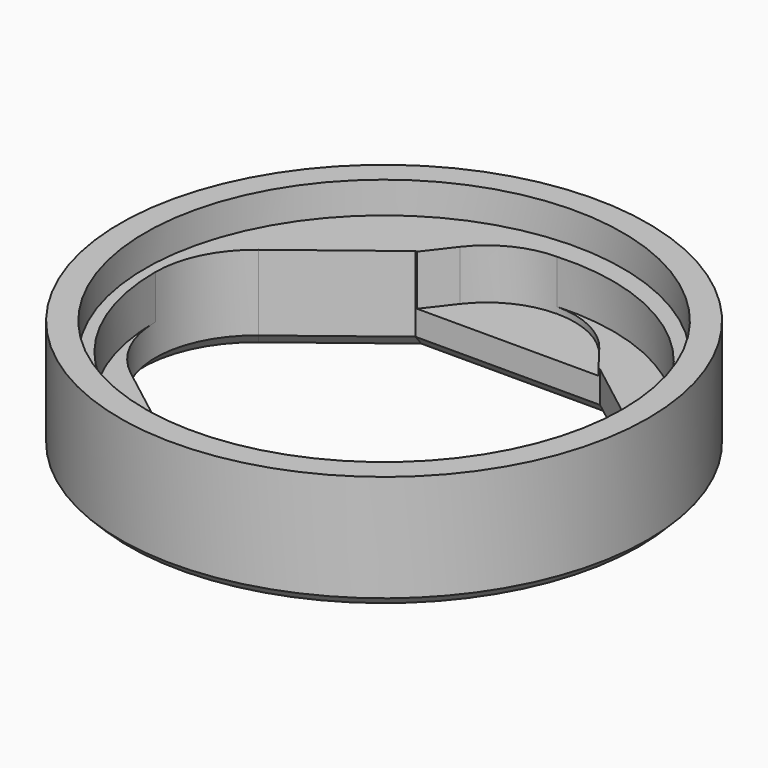
from build123d import *

# Parameters (mm, degrees)
F0_R         = 21
F1_DEPTH     = 3
F2_R         = 21
F3_DEPTH     = 0.5
F4_R         = 21
F5_DEPTH     = 3.5
F6_R         = 21
F6_R_2       = 19
F7_DEPTH     = 2.5
F8_SIZE      = 1
F9_T6_DEPTH  = 12.3424053326
F9_T11_DEPTH = 19.8242698458
F9_T17_DEPTH = 12.3424053326
F9_T20_ANGLE = 104.7950367117
F9_T24_DEPTH = 12.3424053326
F9_T29_DEPTH = 19.8242698458
F9_T35_DEPTH = 12.3424053326
F9_T38_ANGLE = 104.7950367117
F9_T43_DEPTH = 12.3424053326
F9_T47_DEPTH = 19.8242698458
F9_T54_DEPTH = 19.8242698458
F9_T58_DEPTH = 12.3424053326
F9_T65_DEPTH = 12.3424053326
F9_T69_DEPTH = 19.8242698458
F9_T76_DEPTH = 19.8242698458
F9_T80_DEPTH = 12.3424053326


# Not quite as in the source:
# - a fillet or chamfer that OpenCascade refuses, or shapes differently, is made with other operations: its cross-section is extruded or revolved along the edge and cut away or added


with BuildPart() as f1:
    # F0 (on Top) → F1 (new body)
    with BuildSketch(Plane.XY):
        Circle(F0_R)
        with BuildLine():
            Line((-15.0814358373, 6.3381057238), (-7.340451935, 12.3))
            Line((-7.340451935, 12.3), (7.340451935, 12.3))
            Line((7.340451935, 12.3), (15.0814358373, 6.3381057238))
            ThreePointArc((15.0814358373, 6.3381057238), (18.2, 0), (15.0814358373, -6.3381057238))
            Line((15.0814358373, -6.3381057238), (7.340451935, -12.3))
            Line((7.340451935, -12.3), (-7.340451935, -12.3))
            Line((-7.340451935, -12.3), (-15.0814358373, -6.3381057238))
            ThreePointArc((-15.0814358373, -6.3381057238), (-18.2, 0), (-15.0814358373, 6.3381057238))
        make_face(mode=Mode.SUBTRACT)
    extrude(amount=F1_DEPTH)

    # F2 (on face) → F3 (join)
    with BuildSketch(Plane.XY.offset(3)):
        Circle(F2_R)
        with BuildLine():
            Line((-15.0814358373, 6.3381057238), (-7.340451935, 12.3))
            Line((-7.340451935, 12.3), (-7.2180848246, 12.3))
            Line((-7.2180848246, 12.3), (-5.5458425084, 14.4712563576))
            ThreePointArc((-5.5458425084, 14.4712563576), (-3.0904049489, 16.4808755163), (0, 17.2))
            ThreePointArc((0, 17.2), (3.0904049489, 16.4808755163), (5.5458425084, 14.4712563576))
            Line((5.5458425084, 14.4712563576), (7.2180848246, 12.3))
            Line((7.2180848246, 12.3), (7.340451935, 12.3))
            Line((7.340451935, 12.3), (15.0814358373, 6.3381057238))
            ThreePointArc((15.0814358373, 6.3381057238), (17.3781434472, 3.5318913702), (18.2, 0))
            ThreePointArc((18.2, 0), (17.3781434472, -3.5318913702), (15.0814358373, -6.3381057238))
            Line((15.0814358373, -6.3381057238), (7.340451935, -12.3))
            Line((7.340451935, -12.3), (7.2180848246, -12.3))
            Line((7.2180848246, -12.3), (5.5458425084, -14.4712563576))
            ThreePointArc((5.5458425084, -14.4712563576), (3.0904049489, -16.4808755163), (0, -17.2))
            ThreePointArc((0, -17.2), (-3.0904049489, -16.4808755163), (-5.5458425084, -14.4712563576))
            Line((-5.5458425084, -14.4712563576), (-7.2180848246, -12.3))
            Line((-7.2180848246, -12.3), (-7.340451935, -12.3))
            Line((-7.340451935, -12.3), (-15.0814358373, -6.3381057238))
            ThreePointArc((-15.0814358373, -6.3381057238), (-17.3781434472, -3.5318913702), (-18.2, 0))
            ThreePointArc((-18.2, 0), (-17.3781434472, 3.5318913702), (-15.0814358373, 6.3381057238))
        make_face(mode=Mode.SUBTRACT)
    extrude(amount=F3_DEPTH)

    # F4 (on face) → F5 (join)
    with BuildSketch(Plane.XY.offset(3.5)):
        Circle(F4_R)
        with BuildLine():
            Line((-15.0814358373, 6.3381057238), (-7.340451935, 12.3))
            Line((-7.340451935, 12.3), (-7.2180848246, 12.3))
            Line((-7.2180848246, 12.3), (-5.5458425084, 14.4712563576))
            ThreePointArc((-5.5458425084, 14.4712563576), (-3.0904049489, 16.4808755163), (0, 17.2))
            ThreePointArc((0, 17.2), (12.8139825122, 12.529911728), (18.2, 0))
            ThreePointArc((18.2, 0), (17.3781434472, -3.5318913702), (15.0814358373, -6.3381057238))
            Line((15.0814358373, -6.3381057238), (7.340451935, -12.3))
            Line((7.340451935, -12.3), (7.2180848246, -12.3))
            Line((7.2180848246, -12.3), (5.5458425084, -14.4712563576))
            ThreePointArc((5.5458425084, -14.4712563576), (3.0904049489, -16.4808755163), (0, -17.2))
            ThreePointArc((0, -17.2), (-12.8139825122, -12.529911728), (-18.2, 0))
            ThreePointArc((-18.2, 0), (-17.3781434472, 3.5318913702), (-15.0814358373, 6.3381057238))
        make_face(mode=Mode.SUBTRACT)
    extrude(amount=F5_DEPTH)

    # F6 (on face) → F7 (join)
    with BuildSketch(Plane.XY.offset(7)):
        Circle(F6_R)
        Circle(F6_R_2, mode=Mode.SUBTRACT)
    extrude(amount=F7_DEPTH)

    # F8
    f8_edges = [f1.edges().sort_by_distance(p)[0] for p in [
        (-21, 0, 0),
    ]]
    chamfer(f8_edges, length=F8_SIZE)

    # F9: chamfer of 1 on 9 edges, made by hand

    # F9_s1 → F9_t2 (revolve, cut)
    with BuildSketch(Plane.XZ):
        Polygon((20.2928932188, 0.2928932188), (19.5857864376, 0), (20, 0), align=None)
    revolve(axis=Axis((0, 0, 0), (0, 0, 1)), mode=Mode.SUBTRACT)


with BuildPart() as f9_tool4:
    # F9_s5 → F9_t6 (new body)
    with BuildSketch(Plane(origin=(-6.4023462265, -4.9309121171, 0), x_dir=(0, 0, 1), z_dir=(0.7922632155, 0.6101794797, 0))):
        Polygon((0, -15.2238306925), (1, -14.2238306925), (0, -14.2238306925), align=None)
    extrude(amount=F9_T6_DEPTH)

    split(bisect_by=Plane.XZ.offset(-12.3), keep=Keep.TOP)


with BuildPart() as f1_1:
    add(f1.part)

    # F9_t3: cut F9_tool4
    add(f9_tool4.part, mode=Mode.SUBTRACT)


with BuildPart() as f9_tool9:
    # F9_s10 → F9_t11 (new body)
    with BuildSketch(Plane.YZ.offset(-9.9121349229)):
        Polygon((13.3, 0), (12.3, 1), (12.3, 0), align=None)
    extrude(amount=F9_T11_DEPTH)

    split(bisect_by=Plane(origin=(-8.6790896108, 11.2690178409, 0), x_dir=(0, 0, 1), z_dir=(0.6101794797, -0.7922632155, 0)), keep=Keep.TOP)

    split(bisect_by=Plane(origin=(8.6790896108, 11.2690178409, 0), x_dir=(0, 0, 1), z_dir=(-0.6101794797, -0.7922632155, 0)), keep=Keep.TOP)


with BuildPart() as f1_2:
    add(f1_1.part)

    # F9_t8: cut F9_tool9
    add(f9_tool9.part, mode=Mode.SUBTRACT)


with BuildPart() as f9_tool15:
    # F9_s16 → F9_t17 (new body)
    with BuildSketch(Plane(origin=(-3.376087509, 2.6001703465, 0), x_dir=(0, 0, 1), z_dir=(0.7922632155, -0.6101794797, 0))):
        Polygon((0, -15.2238306925), (1, -14.2238306925), (0, -14.2238306925), align=None)
    extrude(amount=F9_T17_DEPTH)

    split(bisect_by=Plane.XZ.offset(-12.3), keep=Keep.TOP)


with BuildPart() as f1_3:
    add(f1_2.part)

    # F9_t14: cut F9_tool15
    add(f9_tool15.part, mode=Mode.SUBTRACT)

    # F9_s19 → F9_t20 (revolve, cut)
    with BuildSketch(Plane(origin=(6.4023462265, -4.9309121171, 0), x_dir=(0, 0, 1), z_dir=(-0.7922632155, 0.6101794797, 0))):
        Polygon((0, 15.2238306925), (1, 14.2238306925), (0, 14.2238306925), align=None)
    revolve(axis=Axis((10.2, 0, 0), (0, 0, -1)), revolution_arc=F9_T20_ANGLE, mode=Mode.SUBTRACT)


with BuildPart() as f9_tool22:
    # F9_s23 → F9_t24 (new body)
    with BuildSketch(Plane(origin=(6.4023462265, 4.9309121171, 0), x_dir=(0, 0, 1), z_dir=(-0.7922632155, -0.6101794797, 0))):
        Polygon((0, -15.2238306925), (1, -14.2238306925), (0, -14.2238306925), align=None)
    extrude(amount=F9_T24_DEPTH)

    split(bisect_by=Plane.XZ.offset(12.3), keep=Keep.BOTTOM)


with BuildPart() as f1_4:
    add(f1_3.part)

    # F9_t21: cut F9_tool22
    add(f9_tool22.part, mode=Mode.SUBTRACT)


with BuildPart() as f9_tool27:
    # F9_s28 → F9_t29 (new body)
    with BuildSketch(Plane.YZ.offset(9.9121349229)):
        Polygon((-13.3, 0), (-12.3, 1), (-12.3, 0), align=None)
    extrude(amount=-F9_T29_DEPTH)

    split(bisect_by=Plane(origin=(8.6790896108, -11.2690178409, 0), x_dir=(0, 0, 1), z_dir=(-0.6101794797, 0.7922632155, 0)), keep=Keep.TOP)

    split(bisect_by=Plane(origin=(-8.6790896108, -11.2690178409, 0), x_dir=(0, 0, 1), z_dir=(0.6101794797, 0.7922632155, 0)), keep=Keep.TOP)


with BuildPart() as f1_5:
    add(f1_4.part)

    # F9_t26: cut F9_tool27
    add(f9_tool27.part, mode=Mode.SUBTRACT)


with BuildPart() as f9_tool33:
    # F9_s34 → F9_t35 (new body)
    with BuildSketch(Plane(origin=(3.376087509, -2.6001703465, 0), x_dir=(0, 0, 1), z_dir=(-0.7922632155, 0.6101794797, 0))):
        Polygon((0, -15.2238306925), (1, -14.2238306925), (0, -14.2238306925), align=None)
    extrude(amount=F9_T35_DEPTH)

    split(bisect_by=Plane.XZ.offset(12.3), keep=Keep.BOTTOM)


with BuildPart() as f1_6:
    add(f1_5.part)

    # F9_t32: cut F9_tool33
    add(f9_tool33.part, mode=Mode.SUBTRACT)

    # F9_s37 → F9_t38 (revolve, cut)
    with BuildSketch(Plane(origin=(-6.4023462265, 4.9309121171, 0), x_dir=(0, 0, 1), z_dir=(0.7922632155, -0.6101794797, 0))):
        Polygon((0, 15.2238306925), (1, 14.2238306925), (0, 14.2238306925), align=None)
    revolve(axis=Axis((-10.2, 0, 0), (0, 0, -1)), revolution_arc=F9_T38_ANGLE, mode=Mode.SUBTRACT)


with BuildPart() as f9_tool41:
    # F9_s42 → F9_t43 (new body)
    with BuildSketch(Plane(origin=(-6.4023462265, -4.9309121171, 0), x_dir=(0, 0, 1), z_dir=(0.7922632155, 0.6101794797, 0))):
        Polygon((0, -15.2238306925), (1, -14.2238306925), (0, -14.2238306925), align=None)
    extrude(amount=F9_T43_DEPTH)

    split(bisect_by=Plane.XZ.offset(-12.3), keep=Keep.BOTTOM)


with BuildPart() as f9_tool45:
    # F9_s46 → F9_t47 (new body)
    with BuildSketch(Plane.YZ.offset(-9.9121349229)):
        Polygon((13.3, 0), (12.3, 1), (12.3, 0), align=None)
    extrude(amount=F9_T47_DEPTH)

    split(bisect_by=Plane(origin=(-8.6790896108, 11.2690178409, 0), x_dir=(0, 0, 1), z_dir=(-0.6101794797, 0.7922632155, 0)), keep=Keep.TOP)


with BuildPart() as f9_tool41_1:
    add(f9_tool41.part)

    # F9_t49: intersect F9_tool45
    add(f9_tool45.part, mode=Mode.INTERSECT)


with BuildPart() as f1_7:
    add(f1_6.part)

    # F9_t39: cut F9_tool41
    add(f9_tool41_1.part, mode=Mode.SUBTRACT)


with BuildPart() as f9_tool52:
    # F9_s53 → F9_t54 (new body)
    with BuildSketch(Plane.YZ.offset(-9.9121349229)):
        Polygon((13.3, 0), (12.3, 1), (12.3, 0), align=None)
    extrude(amount=F9_T54_DEPTH)

    split(bisect_by=Plane(origin=(8.6790896108, 11.2690178409, 0), x_dir=(0, 0, 1), z_dir=(0.6101794797, 0.7922632155, 0)), keep=Keep.TOP)


with BuildPart() as f9_tool56:
    # F9_s57 → F9_t58 (new body)
    with BuildSketch(Plane(origin=(-3.376087509, 2.6001703465, 0), x_dir=(0, 0, 1), z_dir=(0.7922632155, -0.6101794797, 0))):
        Polygon((0, -15.2238306925), (1, -14.2238306925), (0, -14.2238306925), align=None)
    extrude(amount=F9_T58_DEPTH)

    split(bisect_by=Plane.XZ.offset(-12.3), keep=Keep.BOTTOM)


with BuildPart() as f9_tool52_1:
    add(f9_tool52.part)

    # F9_t60: intersect F9_tool56
    add(f9_tool56.part, mode=Mode.INTERSECT)


with BuildPart() as f1_8:
    add(f1_7.part)

    # F9_t50: cut F9_tool52
    add(f9_tool52_1.part, mode=Mode.SUBTRACT)


with BuildPart() as f9_tool63:
    # F9_s64 → F9_t65 (new body)
    with BuildSketch(Plane(origin=(6.4023462265, 4.9309121171, 0), x_dir=(0, 0, 1), z_dir=(-0.7922632155, -0.6101794797, 0))):
        Polygon((0, -15.2238306925), (1, -14.2238306925), (0, -14.2238306925), align=None)
    extrude(amount=F9_T65_DEPTH)

    split(bisect_by=Plane.XZ.offset(12.3), keep=Keep.TOP)


with BuildPart() as f9_tool67:
    # F9_s68 → F9_t69 (new body)
    with BuildSketch(Plane.YZ.offset(9.9121349229)):
        Polygon((-13.3, 0), (-12.3, 1), (-12.3, 0), align=None)
    extrude(amount=-F9_T69_DEPTH)

    split(bisect_by=Plane(origin=(8.6790896108, -11.2690178409, 0), x_dir=(0, 0, 1), z_dir=(0.6101794797, -0.7922632155, 0)), keep=Keep.TOP)


with BuildPart() as f9_tool63_1:
    add(f9_tool63.part)

    # F9_t71: intersect F9_tool67
    add(f9_tool67.part, mode=Mode.INTERSECT)


with BuildPart() as f1_9:
    add(f1_8.part)

    # F9_t61: cut F9_tool63
    add(f9_tool63_1.part, mode=Mode.SUBTRACT)


with BuildPart() as f9_tool74:
    # F9_s75 → F9_t76 (new body)
    with BuildSketch(Plane.YZ.offset(9.9121349229)):
        Polygon((-13.3, 0), (-12.3, 1), (-12.3, 0), align=None)
    extrude(amount=-F9_T76_DEPTH)

    split(bisect_by=Plane(origin=(-8.6790896108, -11.2690178409, 0), x_dir=(0, 0, 1), z_dir=(-0.6101794797, -0.7922632155, 0)), keep=Keep.TOP)


with BuildPart() as f9_tool78:
    # F9_s79 → F9_t80 (new body)
    with BuildSketch(Plane(origin=(3.376087509, -2.6001703465, 0), x_dir=(0, 0, 1), z_dir=(-0.7922632155, 0.6101794797, 0))):
        Polygon((0, -15.2238306925), (1, -14.2238306925), (0, -14.2238306925), align=None)
    extrude(amount=F9_T80_DEPTH)

    split(bisect_by=Plane.XZ.offset(12.3), keep=Keep.TOP)


with BuildPart() as f9_tool74_1:
    add(f9_tool74.part)

    # F9_t82: intersect F9_tool78
    add(f9_tool78.part, mode=Mode.INTERSECT)


with BuildPart() as f1_10:
    add(f1_9.part)

    # F9_t72: cut F9_tool74
    add(f9_tool74_1.part, mode=Mode.SUBTRACT)


solid = f1_10.part
